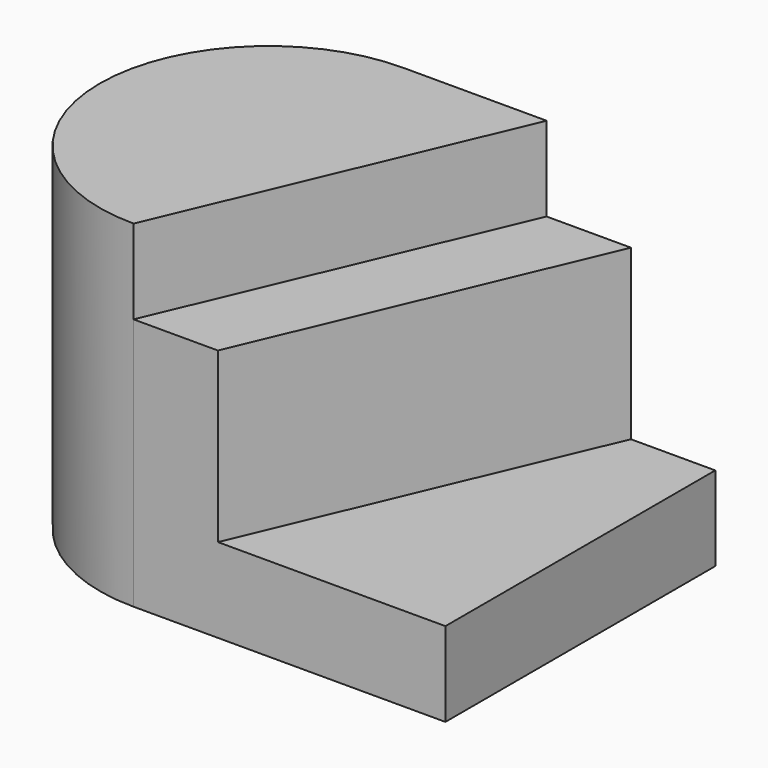
from build123d import *

# Parameters (mm, degrees)
F0_W     = 60
F0_H     = 40
F1_DEPTH = 40
F3_DEPTH = 40
F5_DEPTH = 30
F7_DEPTH = 10


# Not quite as in the source:
# - ends of sketch curves that miss each other by under 0.0002 mm in the source are joined


with BuildPart() as f1:
    # F0 (on Front) → F1 (new body)
    with BuildSketch(Plane.XZ):
        with Locations((30, 20)):
            Rectangle(F0_W, F0_H)
    extrude(amount=F1_DEPTH)

    # F2 (on face) → F3 (cut)
    with BuildSketch(Plane.XY.offset(40)):
        with BuildLine():
            ThreePointArc((23.0189793024, -40), (3.0189805751, -19.9999993636), (23.0189805751, 0))
            Line((23.0189805751, 0), (0, 0))
            Line((0, 0), (0, -40))
            Line((0, -40), (23.0189793024, -40))
        make_face()
    extrude(amount=-F3_DEPTH, mode=Mode.SUBTRACT)

    # F4 (on face) → F5 (cut)
    with BuildSketch(Plane.XY.offset(40)):
        Polygon((50, 0), (33.0189805751, -40), (60, -40), (60, 0), align=None)
    extrude(amount=-F5_DEPTH, mode=Mode.SUBTRACT)

    # F6 (on face) → F7 (cut)
    with BuildSketch(Plane.XY.offset(40)):
        Polygon((40, 0), (23.0189805751, -40), (33.0189805751, -40), (50, 0), align=None)
    extrude(amount=-F7_DEPTH, mode=Mode.SUBTRACT)


solid = f1.part
